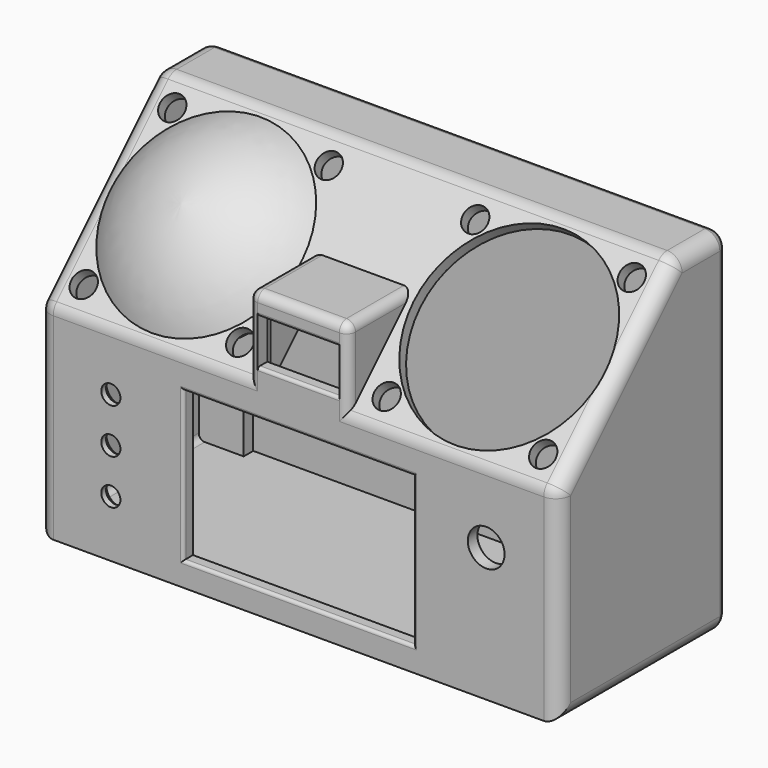
from build123d import *

# Parameters (mm, degrees)
F2_W            = 77
F2_H            = 50
F2_R            = 6.1502507452
F2_W_2          = 27.3
F2_H_2          = 15
F3_DEPTH        = 4
F4_D            = 6.4
F4_CBORE_D      = 9.4
F4_CBORE_DEPTH  = 2
F6_W            = 70.35
F6_H            = 70
F6_R            = 32
F7_W            = 70.35
F7_H            = 70
F7_R            = 32
F8_DEPTH        = 4
F10_DEPTH       = 4
F12_DEPTH       = 4
F13_W           = 33.3
F13_H           = 31.8162338159
F14_DEPTH       = 4
F16_D           = 4.2
F16_CBORE_D     = 8.25
F16_CBORE_DEPTH = 4
F21_W           = 25.3
F21_H           = 26
F22_DEPTH       = 4
F23_W           = 2.8284271247
F23_H           = 2.8284271247
F24_DEPTH       = 174
F25_W           = 174
F25_H           = 117.4974746831
F25_W_2         = 168
F25_H_2         = 111.6690475583
F26_DEPTH       = 15
F27_W           = 15
F27_H           = 15
F28_DEPTH       = 4
F30_DEPTH       = 4
F31_T1_DEPTH    = 65.8578643763
F31_T3_DEPTH    = 78.4289321881
F31_T5_DEPTH    = 92.3259018078
F31_T7_DEPTH    = 65.8578643763
F31_T9_DEPTH    = 65.35
F31_T11_DEPTH   = 65.35
F31_T13_DEPTH   = 164
F31_T15_DEPTH   = 28.2573593129
F31_T20_DEPTH   = 5
F31_T26_DEPTH   = 5
F31_T32_DEPTH   = 5
F31_T38_DEPTH   = 5
F31_2_T1_DEPTH  = 107.4974746831
F31_2_T3_DEPTH  = 164
F31_2_T6_ANGLE  = 90
F31_2_T8_ANGLE  = 90
F31_2_T10_ANGLE = 90
F31_2_T12_ANGLE = 90
F32_R           = 2.99999
F33_T1_DEPTH    = 50
F33_T3_DEPTH    = 77
F33_T5_DEPTH    = 27.3
F33_T11_DEPTH   = 79.5
F33_T15_DEPTH   = 52.5
F33_T22_DEPTH   = 79.5
F33_T26_DEPTH   = 52.5
F33_T33_DEPTH   = 79.5
F33_T37_DEPTH   = 52.5
F33_T44_DEPTH   = 52.5
F33_T48_DEPTH   = 79.5
F34_R           = 2


# Not quite as in the source:
# - a fillet or chamfer that OpenCascade refuses, or shapes differently, is made with other operations: its cross-section is extruded or revolved along the edge and cut away or added
# - a fillet or chamfer is up to 0.001 mm smaller than in the source, because OpenCascade refuses the exact size


with BuildPart() as f3:
    # F2 (on Front) → F3 (new body)
    with BuildSketch(Plane.XZ):
        Polygon((-87, -34), (87, -34), (87, 34), (16.65, 34), (16.65, 61), (-16.65, 61), (-16.65, 34), (-87, 34), align=None)
        with Locations((0, -1)):
            Rectangle(F2_W, F2_H, mode=Mode.SUBTRACT)
        with Locations((62.75, 10.7381668814)):
            Circle(F2_R, mode=Mode.SUBTRACT)
        with Locations((0, 46.5)):
            Rectangle(F2_W_2, F2_H_2, mode=Mode.SUBTRACT)
    extrude(amount=F3_DEPTH)

    # F4 (through all)
    with Locations(Plane(origin=(0, 0, 0), x_dir=(1, 0, 0), z_dir=(0, 1, 0))):
        with Locations((-62.75, 15), (-62.75, 0), (-62.75, -15)):
            CounterBoreHole(F4_D / 2, F4_CBORE_D / 2, F4_CBORE_DEPTH)

    # F6 (on face) + F7 (on face) → F8 (join)
    with BuildSketch(Plane(origin=(0, -19, 19), x_dir=(-1, 0, 0), z_dir=(0, 0.7071067812, -0.7071067812))):
        with Locations((-51.825, 56.2132034356)):
            Rectangle(F6_W, F6_H)
        with Locations((-50.65, 56.2132034356)):
            Circle(F6_R, mode=Mode.SUBTRACT)
    with BuildSketch(Plane(origin=(0, -19, 19), x_dir=(-1, 0, 0), z_dir=(0, 0.7071067812, -0.7071067812))):
        with Locations((51.825, 56.2132034356)):
            Rectangle(F7_W, F7_H)
        with Locations((50.65, 56.2132034356)):
            Circle(F7_R, mode=Mode.SUBTRACT)
    extrude(amount=F8_DEPTH)

    # F9 (on face) → F10 (join)
    with BuildSketch(Plane(origin=(-16.65, 0, 0), x_dir=(0, -1, 0), z_dir=(-1, 0, 0))):
        Polygon((0, 32.3431457505), (0, 61), (-28.6568542495, 61), align=None)
    extrude(amount=-F10_DEPTH)

    # F11 (on face) → F12 (join)
    with BuildSketch(Plane.YZ.offset(16.65)):
        Polygon((28.6568542495, 61), (0, 61), (0, 32.3431457505), align=None)
    extrude(amount=-F12_DEPTH)

    # F13 (on face) → F14 (join)
    with BuildSketch(Plane(origin=(0, -19, 19), x_dir=(1, 0, 0), z_dir=(0, -0.7071067812, 0.7071067812))):
        with Locations((0, 75.3050865276)):
            Rectangle(F13_W, F13_H)
    extrude(amount=-F14_DEPTH)

    # F16 (through all)
    with Locations(Plane(origin=(0, -19, 19), x_dir=(1, 0, 0), z_dir=(0, -0.7071067812, 0.7071067812))):
        with Locations((-76.8129509039, 82.3761543395), (-76.8129509039, 30.0502525317), (-24.4870490961, 82.3761543395), (-24.4870490961, 30.0502525317), (24.4870490961, 30.0502525317), (24.4870490961, 82.3761543395), (76.8129509039, 82.3761543395), (76.8129509039, 30.0502525317)):
            CounterBoreHole(F16_D / 2, F16_CBORE_D / 2, F16_CBORE_DEPTH)

    # F17 (on face) → F20 section 0
    with BuildSketch(Plane.XZ):
        Polygon((87, -34), (87, 32.3431457505), (84, 32.3431457505), (84, -31), (-84, -31), (-84, 32.3431457505), (-87, 32.3431457505), (-87, -34), align=None)
    # F19 (on face) → F20 section 1
    with BuildSketch(Plane(origin=(0, 48.3259018078, 0), x_dir=(-1, 0, 0), z_dir=(0, 1, 0))):
        Polygon((-84, 83.4974746831), (-87, 83.4974746831), (-87, -34), (87, -34), (87, 83.4974746831), (84, 83.4974746831), (84, -31), (-84, -31), align=None)
    loft()

    # F21 (on face) → F22 (join)
    with BuildSketch(Plane.XY.offset(61)):
        with Locations((0, 13)):
            Rectangle(F21_W, F21_H)
    extrude(amount=-F22_DEPTH)

    # F23 (on face) → F24 (join, through all)
    with BuildSketch(Plane(origin=(-87, 0, 0), x_dir=(0, -1, 0), z_dir=(-1, 0, 0))):
        with Locations((-46.9116882454, 82.0832611207)):
            Rectangle(F23_W, F23_H)
    extrude(amount=-F24_DEPTH)

    # F25 (on face) → F26 (join)
    with BuildSketch(Plane(origin=(0, 48.3259018078, 0), x_dir=(-1, 0, 0), z_dir=(0, 1, 0))):
        with Locations((0, 24.7487373415)):
            Rectangle(F25_W, F25_H)
        with Locations((0, 24.8345237792)):
            Rectangle(F25_W_2, F25_H_2, mode=Mode.SUBTRACT)
    extrude(amount=F26_DEPTH)

    # F27 (on face) → F28 (join)
    with BuildSketch(Plane(origin=(0, 63.3259018078, 0), x_dir=(-1, 0, 0), z_dir=(0, 1, 0))):
        with Locations((-76.5, 73.1690475583)):
            Rectangle(F27_W, F27_H)
        with Locations((-76.5, -23.5)):
            Rectangle(F27_W, F27_H)
        with Locations((76.5, -23.5)):
            Rectangle(F27_W, F27_H)
        with Locations((76.5, 73.1690475583)):
            Rectangle(F27_W, F27_H)
    extrude(amount=-F28_DEPTH)

    # F31: fillet of radius 5 on 11 edges, made by hand

    # F31_s2 → F31_t1 (cut)
    with BuildSketch(Plane(origin=(0, 16.4644660941, 16.4644660941), x_dir=(1, 0, 0), z_dir=(0, 0.7071067812, 0.7071067812))):
        with BuildLine():
            ThreePointArc((-87, -21.8700576851), (-85.5355339059, -25.405591591), (-82, -26.8700576851))
            Line((-82, -26.8700576851), (-87, -26.8700576851))
            Line((-87, -26.8700576851), (-87, -21.8700576851))
        make_face()
    extrude(amount=F31_T1_DEPTH, mode=Mode.SUBTRACT)

    # F31_s4 → F31_t3 (cut)
    with BuildSketch(Plane.XY.offset(-46.5)):
        with BuildLine():
            ThreePointArc((-87, 1), (-85.5355339059, -2.5355339059), (-82, -4))
            Line((-82, -4), (-87, -4))
            Line((-87, -4), (-87, 1))
        make_face()
        with BuildLine():
            ThreePointArc((82, -4), (85.5355339059, -2.5355339059), (87, 1))
            Line((87, 1), (87, -4))
            Line((87, -4), (82, -4))
        make_face()
    extrude(amount=F31_T3_DEPTH, mode=Mode.SUBTRACT)

    # F31_s6 → F31_t5 (cut)
    with BuildSketch(Plane.XZ.offset(-75.8259018078)):
        with BuildLine():
            ThreePointArc((-87, -29), (-85.5355339059, -32.5355339059), (-82, -34))
            Line((-82, -34), (-87, -34))
            Line((-87, -34), (-87, -29))
        make_face()
        with BuildLine():
            ThreePointArc((82, -34), (85.5355339059, -32.5355339059), (87, -29))
            Line((87, -29), (87, -34))
            Line((87, -34), (82, -34))
        make_face()
    extrude(amount=F31_T5_DEPTH, mode=Mode.SUBTRACT)

    # F31_s8 → F31_t7 (cut)
    with BuildSketch(Plane(origin=(0, 63.033008589, 63.033008589), x_dir=(1, 0, 0), z_dir=(0, -0.7071067812, -0.7071067812))):
        with BuildLine():
            ThreePointArc((82, 26.8700576851), (85.5355339059, 25.405591591), (87, 21.8700576851))
            Line((87, 21.8700576851), (87, 26.8700576851))
            Line((87, 26.8700576851), (82, 26.8700576851))
        make_face()
    extrude(amount=F31_T7_DEPTH, mode=Mode.SUBTRACT)

    # F31_s10 → F31_t9 (cut)
    with BuildSketch(Plane.YZ.offset(-82)):
        with BuildLine():
            ThreePointArc((-2.5355339059, 35.4644660941), (-3.6193976626, 33.84234935), (-4, 31.9289321881))
            Line((-4, 31.9289321881), (-4, 34))
            Line((-4, 34), (-2.5355339059, 35.4644660941))
        make_face()
    extrude(amount=F31_T9_DEPTH, mode=Mode.SUBTRACT)

    # F31_s12 → F31_t11 (cut)
    with BuildSketch(Plane.YZ.offset(16.65)):
        with BuildLine():
            ThreePointArc((-2.5355339059, 35.4644660941), (-3.6193976626, 33.84234935), (-4, 31.9289321881))
            Line((-4, 31.9289321881), (-4, 34))
            Line((-4, 34), (-2.5355339059, 35.4644660941))
        make_face()
    extrude(amount=F31_T11_DEPTH, mode=Mode.SUBTRACT)

    # F31_s14 → F31_t13 (cut)
    with BuildSketch(Plane.YZ.offset(-82)):
        with BuildLine():
            ThreePointArc((44.033008589, 82.033008589), (45.6551253331, 83.1168723456), (47.5685424949, 83.4974746831))
            Line((47.5685424949, 83.4974746831), (45.4974746831, 83.4974746831))
            Line((45.4974746831, 83.4974746831), (44.033008589, 82.033008589))
        make_face()
    extrude(amount=F31_T13_DEPTH, mode=Mode.SUBTRACT)

    # F31_s16 → F31_t15 (cut)
    with BuildSketch(Plane.XZ.offset(-75.8259018078)):
        with BuildLine():
            ThreePointArc((82, 83.4974746831), (85.5355339059, 82.033008589), (87, 78.4974746831))
            Line((87, 78.4974746831), (87, 83.4974746831))
            Line((87, 83.4974746831), (82, 83.4974746831))
        make_face()
        with BuildLine():
            ThreePointArc((-87, 78.4974746831), (-85.5355339059, 82.033008589), (-82, 83.4974746831))
            Line((-82, 83.4974746831), (-87, 83.4974746831))
            Line((-87, 83.4974746831), (-87, 78.4974746831))
        make_face()
    extrude(amount=F31_T15_DEPTH, mode=Mode.SUBTRACT)


with BuildPart() as f30:
    # F29 (on face) → F30 (new body)
    with BuildSketch(Plane(origin=(0, 63.3259018078, 0), x_dir=(-1, 0, 0), z_dir=(0, 1, 0))):
        with BuildLine():
            Line((82, 83.4974746831), (-82, 83.4974746831))
            ThreePointArc((-82, 83.4974746831), (-85.5355339059, 82.033008589), (-87, 78.4974746831))
            Line((-87, 78.4974746831), (-87, -29))
            ThreePointArc((-87, -29), (-85.5355339059, -32.5355339059), (-82, -34))
            Line((-82, -34), (82, -34))
            ThreePointArc((82, -34), (85.5355339059, -32.5355339059), (87, -29))
            Line((87, -29), (87, 78.4974746831))
            ThreePointArc((87, 78.4974746831), (85.5355339059, 82.033008589), (82, 83.4974746831))
        make_face()
    extrude(amount=F30_DEPTH)

    # F31#2: fillet of radius 5 on 1 edges, made by hand

    # F31_2_s2 → F31_2_t1 (cut)
    with BuildSketch(Plane.XY.offset(-29)):
        with BuildLine():
            ThreePointArc((87, 63.3259018078), (85.2632981746, 66.198885154), (82.1010205144, 67.3259018078))
            Line((82.1010205144, 67.3259018078), (87, 67.3259018078))
            Line((87, 67.3259018078), (87, 63.3259018078))
        make_face()
        with BuildLine():
            ThreePointArc((-87, 63.3259018078), (-85.2632981746, 66.198885154), (-82.1010205144, 67.3259018078))
            Line((-82.1010205144, 67.3259018078), (-87, 67.3259018078))
            Line((-87, 67.3259018078), (-87, 63.3259018078))
        make_face()
    extrude(amount=F31_2_T1_DEPTH, mode=Mode.SUBTRACT)

    # F31_2_s4 → F31_2_t3 (cut)
    with BuildSketch(Plane.YZ.offset(-82)):
        with BuildLine():
            ThreePointArc((63.3259018078, -34), (66.198885154, -32.2632981746), (67.3259018078, -29.1010205144))
            Line((67.3259018078, -29.1010205144), (67.3259018078, -34))
            Line((67.3259018078, -34), (63.3259018078, -34))
        make_face()
        with BuildLine():
            ThreePointArc((63.3259018078, 83.4974746831), (66.198885154, 81.7607728577), (67.3259018078, 78.5984951975))
            Line((67.3259018078, 78.5984951975), (67.3259018078, 83.4974746831))
            Line((67.3259018078, 83.4974746831), (63.3259018078, 83.4974746831))
        make_face()
    extrude(amount=F31_2_T3_DEPTH, mode=Mode.SUBTRACT)

    # F31_2_s5 → F31_2_t6 (revolve, cut)
    with BuildSketch(Plane.YZ.offset(82)):
        with BuildLine():
            ThreePointArc((63.3259018078, 83.4974746831), (66.198885154, 81.7607728577), (67.3259018078, 78.5984951975))
            Line((67.3259018078, 78.5984951975), (67.3259018078, 83.4974746831))
            Line((67.3259018078, 83.4974746831), (63.3259018078, 83.4974746831))
        make_face()
    revolve(axis=Axis((82, 67.3259018078, 78.4974746831), (0, 1, 0)), revolution_arc=F31_2_T6_ANGLE, mode=Mode.SUBTRACT)

    # F31_2_s7 → F31_2_t8 (revolve, cut)
    with BuildSketch(Plane.XY.offset(-29)):
        with BuildLine():
            ThreePointArc((87, 63.3259018078), (85.2632981746, 66.198885154), (82.1010205144, 67.3259018078))
            Line((82.1010205144, 67.3259018078), (87, 67.3259018078))
            Line((87, 67.3259018078), (87, 63.3259018078))
        make_face()
    revolve(axis=Axis((82, 67.3259018078, -29), (0, 1, 0)), revolution_arc=F31_2_T8_ANGLE, mode=Mode.SUBTRACT)

    # F31_2_s9 → F31_2_t10 (revolve, cut)
    with BuildSketch(Plane.YZ.offset(-82)):
        with BuildLine():
            ThreePointArc((63.3259018078, -34), (66.198885154, -32.2632981746), (67.3259018078, -29.1010205144))
            Line((67.3259018078, -29.1010205144), (67.3259018078, -34))
            Line((67.3259018078, -34), (63.3259018078, -34))
        make_face()
    revolve(axis=Axis((-82, 67.3259018078, -29), (0, 1, 0)), revolution_arc=F31_2_T10_ANGLE, mode=Mode.SUBTRACT)

    # F31_2_s11 → F31_2_t12 (revolve, cut)
    with BuildSketch(Plane.XY.offset(78.4974746831)):
        with BuildLine():
            ThreePointArc((-87, 63.3259018078), (-85.2632981746, 66.198885154), (-82.1010205144, 67.3259018078))
            Line((-82.1010205144, 67.3259018078), (-87, 67.3259018078))
            Line((-87, 67.3259018078), (-87, 63.3259018078))
        make_face()
    revolve(axis=Axis((-82, 67.3259018078, 78.4974746831), (0, 1, 0)), revolution_arc=F31_2_T12_ANGLE, mode=Mode.SUBTRACT)


with BuildPart() as f31_tool18:
    # F31_s19 → F31_t20 (new body)
    with BuildSketch(Plane.YZ.offset(-82)):
        Polygon((1, 31.9289321881), (-2.5355339059, 35.4644660941), (-4, 34), (-4, 31.9289321881), align=None)
    extrude(amount=-F31_T20_DEPTH)

    # F31_s21 → F31_t22 (revolve, cut)
    with BuildSketch(Plane(origin=(-82, 1, 31.9289321881), x_dir=(0, 0.9238795325, -0.3826834324), z_dir=(0, 0.3826834324, 0.9238795325))):
        with BuildLine():
            ThreePointArc((0, -5), (5, 0), (0, 5))
            Line((0, 5), (0, -5))
        make_face()
    revolve(axis=Axis((-82, 1, 31.9289321881), (-1, 0, 0)), mode=Mode.SUBTRACT)


with BuildPart() as f3_1:
    add(f3.part)

    # F31_t17: cut F31_tool18
    add(f31_tool18.part, mode=Mode.SUBTRACT)


with BuildPart() as f31_tool24:
    # F31_s25 → F31_t26 (new body)
    with BuildSketch(Plane.YZ.offset(-82)):
        Polygon((47.5685424949, 78.4974746831), (44.033008589, 82.033008589), (45.4974746831, 83.4974746831), (47.5685424949, 83.4974746831), align=None)
    extrude(amount=-F31_T26_DEPTH)

    # F31_s27 → F31_t28 (revolve, cut)
    with BuildSketch(Plane(origin=(-82, 47.5685424949, 78.4974746831), x_dir=(0, 0.3826834324, -0.9238795325), z_dir=(0, 0.9238795325, 0.3826834324))):
        with BuildLine():
            ThreePointArc((0, -5), (5, 0), (0, 5))
            Line((0, 5), (0, -5))
        make_face()
    revolve(axis=Axis((-82, 47.5685424949, 78.4974746831), (-1, 0, 0)), mode=Mode.SUBTRACT)


with BuildPart() as f3_2:
    add(f3_1.part)

    # F31_t23: cut F31_tool24
    add(f31_tool24.part, mode=Mode.SUBTRACT)


with BuildPart() as f31_tool30:
    # F31_s31 → F31_t32 (new body)
    with BuildSketch(Plane.YZ.offset(82)):
        Polygon((1, 31.9289321881), (-2.5355339059, 35.4644660941), (-4, 34), (-4, 31.9289321881), align=None)
    extrude(amount=F31_T32_DEPTH)

    # F31_s33 → F31_t34 (revolve, cut)
    with BuildSketch(Plane(origin=(82, 1, 31.9289321881), x_dir=(0, 0.9238795325, -0.3826834324), z_dir=(0, -0.3826834324, -0.9238795325))):
        with BuildLine():
            ThreePointArc((0, -5), (5, 0), (0, 5))
            Line((0, 5), (0, -5))
        make_face()
    revolve(axis=Axis((82, 1, 31.9289321881), (1, 0, 0)), mode=Mode.SUBTRACT)


with BuildPart() as f3_3:
    add(f3_2.part)

    # F31_t29: cut F31_tool30
    add(f31_tool30.part, mode=Mode.SUBTRACT)


with BuildPart() as f31_tool36:
    # F31_s37 → F31_t38 (new body)
    with BuildSketch(Plane.YZ.offset(82)):
        Polygon((47.5685424949, 78.4974746831), (44.033008589, 82.033008589), (45.4974746831, 83.4974746831), (47.5685424949, 83.4974746831), align=None)
    extrude(amount=F31_T38_DEPTH)

    # F31_s39 → F31_t40 (revolve, cut)
    with BuildSketch(Plane(origin=(82, 47.5685424949, 78.4974746831), x_dir=(0, 0.3826834324, -0.9238795325), z_dir=(0, -0.9238795325, -0.3826834324))):
        with BuildLine():
            ThreePointArc((0, -5), (5, 0), (0, 5))
            Line((0, 5), (0, -5))
        make_face()
    revolve(axis=Axis((82, 47.5685424949, 78.4974746831), (1, 0, 0)), mode=Mode.SUBTRACT)


with BuildPart() as f3_4:
    add(f3_3.part)

    # F31_t35: cut F31_tool36
    add(f31_tool36.part, mode=Mode.SUBTRACT)

    # F32 (radius 3 in the source; OpenCascade refuses exactly that, so slightly less here)
    f32_edges = [f3_4.edges().sort_by_distance(p)[0] for p in [
        (-16.65, -4, 46.464466),
        (16.65, -4, 46.464466),
        (0, -4, 61),
        (-16.65, 9.5, 61),
        (16.65, 9.5, 61),
    ]]
    fillet(f32_edges, radius=F32_R)

    # F33: fillet of radius 1 on 6 edges, made by hand

    # F33_s2 → F33_t1 (cut)
    with BuildSketch(Plane.XY.offset(-26)):
        with BuildLine():
            ThreePointArc((-39.5, -4), (-38.7928932188, -3.7071067812), (-38.5, -3))
            Line((-38.5, -3), (-38.5, -4))
            Line((-38.5, -4), (-39.5, -4))
        make_face()
        with BuildLine():
            ThreePointArc((39.5, -4), (38.7928932188, -3.7071067812), (38.5, -3))
            Line((38.5, -3), (38.5, -4))
            Line((38.5, -4), (39.5, -4))
        make_face()
    extrude(amount=F33_T1_DEPTH, mode=Mode.SUBTRACT)

    # F33_s4 → F33_t3 (cut)
    with BuildSketch(Plane.YZ.offset(-38.5)):
        with BuildLine():
            ThreePointArc((-4, 25), (-3.7071067812, 24.2928932188), (-3, 24))
            Line((-3, 24), (-4, 24))
            Line((-4, 24), (-4, 25))
        make_face()
        with BuildLine():
            ThreePointArc((-4, -27), (-3.7071067812, -26.2928932188), (-3, -26))
            Line((-3, -26), (-4, -26))
            Line((-4, -26), (-4, -27))
        make_face()
    extrude(amount=F33_T3_DEPTH, mode=Mode.SUBTRACT)

    # F33_s6 → F33_t5 (cut)
    with BuildSketch(Plane.YZ.offset(-13.65)):
        with BuildLine():
            ThreePointArc((-4, 38), (-3.7071067812, 38.7071067812), (-3, 39))
            Line((-3, 39), (-4, 39))
            Line((-4, 39), (-4, 38))
        make_face()
        with BuildLine():
            ThreePointArc((-4, 55), (-3.7071067812, 54.2928932188), (-3, 54))
            Line((-3, 54), (-4, 54))
            Line((-4, 54), (-4, 55))
        make_face()
    extrude(amount=F33_T5_DEPTH, mode=Mode.SUBTRACT)


with BuildPart() as f33_tool9:
    # F33_s10 → F33_t11 (new body)
    with BuildSketch(Plane.YZ.offset(38.5)):
        with BuildLine():
            ThreePointArc((-4, -27), (-3.7071067812, -26.2928932188), (-3, -26))
            Line((-3, -26), (-4, -26))
            Line((-4, -26), (-4, -27))
        make_face()
    extrude(amount=-F33_T11_DEPTH)

    split(bisect_by=Plane.YZ.offset(-38.5), keep=Keep.BOTTOM)


with BuildPart() as f33_tool13:
    # F33_s14 → F33_t15 (new body)
    with BuildSketch(Plane.XY.offset(-28.5)):
        with BuildLine():
            ThreePointArc((-39.5, -4), (-38.7928932188, -3.7071067812), (-38.5, -3))
            Line((-38.5, -3), (-38.5, -4))
            Line((-38.5, -4), (-39.5, -4))
        make_face()
    extrude(amount=F33_T15_DEPTH)

    split(bisect_by=Plane.XY.offset(-26), keep=Keep.BOTTOM)


with BuildPart() as f33_tool9_1:
    add(f33_tool9.part)

    # F33_t17: intersect F33_tool13
    add(f33_tool13.part, mode=Mode.INTERSECT)


with BuildPart() as f3_5:
    add(f3_4.part)

    # F33_t7: cut F33_tool9
    add(f33_tool9_1.part, mode=Mode.SUBTRACT)


with BuildPart() as f33_tool20:
    # F33_s21 → F33_t22 (new body)
    with BuildSketch(Plane.YZ.offset(-41)):
        with BuildLine():
            ThreePointArc((-4, 25), (-3.7071067812, 24.2928932188), (-3, 24))
            Line((-3, 24), (-4, 24))
            Line((-4, 24), (-4, 25))
        make_face()
    extrude(amount=F33_T22_DEPTH)

    split(bisect_by=Plane.YZ.offset(-38.5), keep=Keep.BOTTOM)


with BuildPart() as f33_tool24:
    # F33_s25 → F33_t26 (new body)
    with BuildSketch(Plane.XY.offset(-26)):
        with BuildLine():
            ThreePointArc((-39.5, -4), (-38.7928932188, -3.7071067812), (-38.5, -3))
            Line((-38.5, -3), (-38.5, -4))
            Line((-38.5, -4), (-39.5, -4))
        make_face()
    extrude(amount=F33_T26_DEPTH)

    split(bisect_by=Plane.XY.offset(24), keep=Keep.TOP)


with BuildPart() as f33_tool20_1:
    add(f33_tool20.part)

    # F33_t28: intersect F33_tool24
    add(f33_tool24.part, mode=Mode.INTERSECT)


with BuildPart() as f3_6:
    add(f3_5.part)

    # F33_t18: cut F33_tool20
    add(f33_tool20_1.part, mode=Mode.SUBTRACT)


with BuildPart() as f33_tool31:
    # F33_s32 → F33_t33 (new body)
    with BuildSketch(Plane.YZ.offset(-38.5)):
        with BuildLine():
            ThreePointArc((-4, 25), (-3.7071067812, 24.2928932188), (-3, 24))
            Line((-3, 24), (-4, 24))
            Line((-4, 24), (-4, 25))
        make_face()
    extrude(amount=F33_T33_DEPTH)

    split(bisect_by=Plane.YZ.offset(38.5), keep=Keep.TOP)


with BuildPart() as f33_tool35:
    # F33_s36 → F33_t37 (new body)
    with BuildSketch(Plane.XY.offset(26.5)):
        with BuildLine():
            ThreePointArc((39.5, -4), (38.7928932188, -3.7071067812), (38.5, -3))
            Line((38.5, -3), (38.5, -4))
            Line((38.5, -4), (39.5, -4))
        make_face()
    extrude(amount=-F33_T37_DEPTH)

    split(bisect_by=Plane.XY.offset(24), keep=Keep.TOP)


with BuildPart() as f33_tool31_1:
    add(f33_tool31.part)

    # F33_t39: intersect F33_tool35
    add(f33_tool35.part, mode=Mode.INTERSECT)


with BuildPart() as f3_7:
    add(f3_6.part)

    # F33_t29: cut F33_tool31
    add(f33_tool31_1.part, mode=Mode.SUBTRACT)


with BuildPart() as f33_tool42:
    # F33_s43 → F33_t44 (new body)
    with BuildSketch(Plane.XY.offset(24)):
        with BuildLine():
            ThreePointArc((39.5, -4), (38.7928932188, -3.7071067812), (38.5, -3))
            Line((38.5, -3), (38.5, -4))
            Line((38.5, -4), (39.5, -4))
        make_face()
    extrude(amount=-F33_T44_DEPTH)

    split(bisect_by=Plane.XY.offset(-26), keep=Keep.BOTTOM)


with BuildPart() as f33_tool46:
    # F33_s47 → F33_t48 (new body)
    with BuildSketch(Plane.YZ.offset(41)):
        with BuildLine():
            ThreePointArc((-4, -27), (-3.7071067812, -26.2928932188), (-3, -26))
            Line((-3, -26), (-4, -26))
            Line((-4, -26), (-4, -27))
        make_face()
    extrude(amount=-F33_T48_DEPTH)

    split(bisect_by=Plane.YZ.offset(38.5), keep=Keep.TOP)


with BuildPart() as f33_tool42_1:
    add(f33_tool42.part)

    # F33_t50: intersect F33_tool46
    add(f33_tool46.part, mode=Mode.INTERSECT)


with BuildPart() as f3_8:
    add(f3_7.part)

    # F33_t40: cut F33_tool42
    add(f33_tool42_1.part, mode=Mode.SUBTRACT)

    # F34
    f34_edges = [f3_8.edges().sort_by_distance(p)[0] for p in [
        (84, 29.662951, -31),
        (-84, 29.662951, -31),
        (-84, 0, 0.671573),
        (84, 0, 0.671573),
        (48.325, 0, 32.343146),
        (-48.325, 0, 32.343146),
    ]]
    fillet(f34_edges, radius=F34_R)

    # F37 (on plane+point) → F38 (revolve)
    with BuildSketch(Plane.YZ.offset(-50.65)):
        with BuildLine():
            ThreePointArc((10.2394465396, 69.2580281435), (1.1603643401, 53.7940981594), (-1.8786796564, 36.1213203436))
            Line((-1.8786796564, 36.1213203436), (2.3639610307, 31.8786796564))
            ThreePointArc((2.3639610307, 31.8786796564), (4.1831109714, 50.2468166951), (13.0763619852, 66.4211126979))
            Line((13.0763619852, 66.4211126979), (10.2394465396, 69.2580281435))
        make_face()
    revolve(axis=Axis((-50.65, 15.4940919406, 64.0033827425), (0, -0.7071067812, 0.7071067812)))


solid = Compound([f30.part, f3_8.part])
